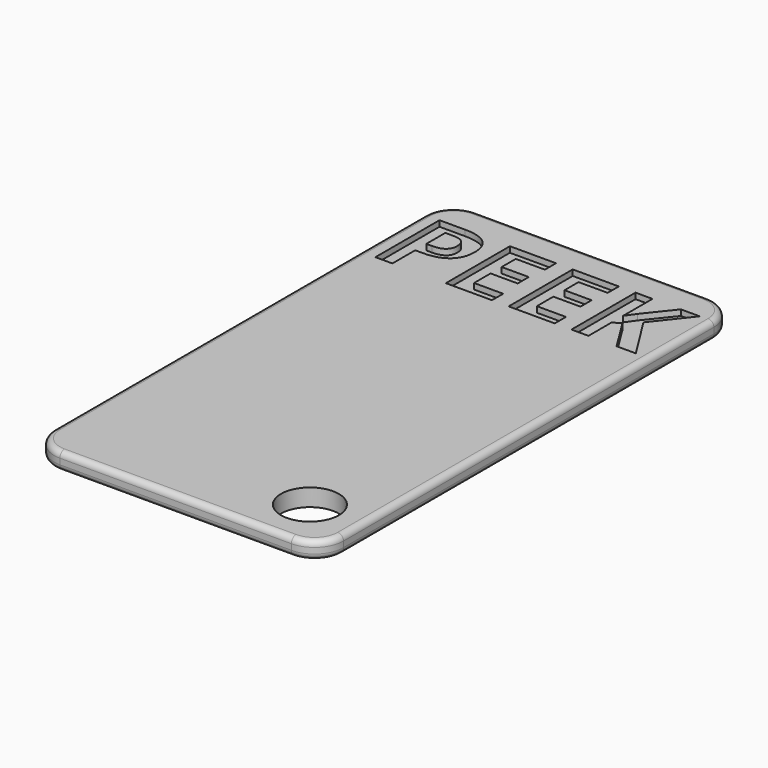
from build123d import *

# Parameters (mm, degrees)
F0_W         = 90
F0_H         = 50
F1_DEPTH     = 3
F2_R         = 1
F3_T1_DEPTH  = 3
F3_T4_ANGLE  = 90
F3_T6_ANGLE  = 90
F3_T8_ANGLE  = 90
F3_T10_ANGLE = 90
F3_T12_ANGLE = 90
F3_T14_ANGLE = 90
F3_T16_ANGLE = 90
F3_T18_ANGLE = 90
F5_ANGLE     = 90
F6_TEXT_SIZE = 19.3792581378
F7_DEPTH     = 1
F8_R         = 5
F9_DEPTH     = 3


# Not quite as in the source:
# - a fillet or chamfer that OpenCascade refuses, or shapes differently, is made with other operations: its cross-section is extruded or revolved along the edge and cut away or added
# - Text() gives the source's letters only with a copy of the font that has no kerning and outlines rounded to 1/6400 em; it was checked with that copy


with BuildPart() as f1:
    # F0 (on Top) → F1 (new body)
    with BuildSketch(Plane.XY):
        Rectangle(F0_W, F0_H)
    extrude(amount=F1_DEPTH)

    # F2
    f2_edges = [f1.edges().sort_by_distance(p)[0] for p in [
        (0, 25, 3),
        (-45, 0, 3),
        (0, -25, 3),
        (45, 0, 3),
        (0, 25, 0),
        (-45, 0, 0),
        (0, -25, 0),
        (45, 0, 0),
    ]]
    fillet(f2_edges, radius=F2_R)

    # F3: fillet of radius 5 on 4 edges, made by hand

    # F3_s2 → F3_t1 (cut)
    with BuildSketch(Plane.XY):
        with BuildLine():
            ThreePointArc((45, -20), (43.5355339059, -23.5355339059), (40, -25))
            Line((40, -25), (45, -25))
            Line((45, -25), (45, -20))
        make_face()
        with BuildLine():
            ThreePointArc((40, 25), (43.5355339059, 23.5355339059), (45, 20))
            Line((45, 20), (45, 25))
            Line((45, 25), (40, 25))
        make_face()
        with BuildLine():
            ThreePointArc((-40, 25), (-43.5355339059, 23.5355339059), (-45, 20))
            Line((-45, 20), (-45, 25))
            Line((-45, 25), (-40, 25))
        make_face()
        with BuildLine():
            ThreePointArc((-45, -20), (-43.5355339059, -23.5355339059), (-40, -25))
            Line((-40, -25), (-45, -25))
            Line((-45, -25), (-45, -20))
        make_face()
    extrude(amount=F3_T1_DEPTH, mode=Mode.SUBTRACT)

    # F3_s3 → F3_t4 (revolve, cut)
    with BuildSketch(Plane.YZ.offset(-40)):
        with BuildLine():
            ThreePointArc((-24, 0), (-24.7071067812, 0.2928932188), (-25, 1))
            Line((-25, 1), (-25, 0))
            Line((-25, 0), (-24, 0))
        make_face()
    revolve(axis=Axis((-40, -20, 0), (0, 0, -1)), revolution_arc=F3_T4_ANGLE, mode=Mode.SUBTRACT)

    # F3_s5 → F3_t6 (revolve, cut)
    with BuildSketch(Plane.XZ.offset(20)):
        with BuildLine():
            ThreePointArc((-44, 3), (-44.7071067812, 2.7071067812), (-45, 2))
            Line((-45, 2), (-45, 3))
            Line((-45, 3), (-44, 3))
        make_face()
    revolve(axis=Axis((-40, -20, 3), (0, 0, 1)), revolution_arc=F3_T6_ANGLE, mode=Mode.SUBTRACT)

    # F3_s7 → F3_t8 (revolve, cut)
    with BuildSketch(Plane.XZ.offset(-20)):
        with BuildLine():
            ThreePointArc((-44, 0), (-44.7071067812, 0.2928932188), (-45, 1))
            Line((-45, 1), (-45, 0))
            Line((-45, 0), (-44, 0))
        make_face()
    revolve(axis=Axis((-40, 20, 0), (0, 0, -1)), revolution_arc=F3_T8_ANGLE, mode=Mode.SUBTRACT)

    # F3_s9 → F3_t10 (revolve, cut)
    with BuildSketch(Plane.YZ.offset(-40)):
        with BuildLine():
            ThreePointArc((24, 3), (24.7071067812, 2.7071067812), (25, 2))
            Line((25, 2), (25, 3))
            Line((25, 3), (24, 3))
        make_face()
    revolve(axis=Axis((-40, 20, 3), (0, 0, 1)), revolution_arc=F3_T10_ANGLE, mode=Mode.SUBTRACT)

    # F3_s11 → F3_t12 (revolve, cut)
    with BuildSketch(Plane.YZ.offset(40)):
        with BuildLine():
            ThreePointArc((24, 0), (24.7071067812, 0.2928932188), (25, 1))
            Line((25, 1), (25, 0))
            Line((25, 0), (24, 0))
        make_face()
    revolve(axis=Axis((40, 20, 0), (0, 0, -1)), revolution_arc=F3_T12_ANGLE, mode=Mode.SUBTRACT)

    # F3_s13 → F3_t14 (revolve, cut)
    with BuildSketch(Plane.XZ.offset(-20)):
        with BuildLine():
            ThreePointArc((44, 3), (44.7071067812, 2.7071067812), (45, 2))
            Line((45, 2), (45, 3))
            Line((45, 3), (44, 3))
        make_face()
    revolve(axis=Axis((40, 20, 3), (0, 0, 1)), revolution_arc=F3_T14_ANGLE, mode=Mode.SUBTRACT)

    # F3_s15 → F3_t16 (revolve, cut)
    with BuildSketch(Plane.XZ.offset(20)):
        with BuildLine():
            ThreePointArc((44, 0), (44.7071067812, 0.2928932188), (45, 1))
            Line((45, 1), (45, 0))
            Line((45, 0), (44, 0))
        make_face()
    revolve(axis=Axis((40, -20, 0), (0, 0, -1)), revolution_arc=F3_T16_ANGLE, mode=Mode.SUBTRACT)

    # F3_s17 → F3_t18 (revolve, cut)
    with BuildSketch(Plane.YZ.offset(40)):
        with BuildLine():
            ThreePointArc((-24, 3), (-24.7071067812, 2.7071067812), (-25, 2))
            Line((-25, 2), (-25, 3))
            Line((-25, 3), (-24, 3))
        make_face()
    revolve(axis=Axis((40, -20, 3), (0, 0, 1)), revolution_arc=F3_T18_ANGLE, mode=Mode.SUBTRACT)


with BuildPart() as f1_1:
    # F5: moved
    add(f1.part.rotate(Axis((0, 0, 16.4477843791), (0, 0, 1)), F5_ANGLE))

    # F6 (on face) → F7 (cut)
    with BuildSketch(Plane.XY.offset(3)):
        with Locations((-24, 25.9722985371)):
            Text('PEEK', F6_TEXT_SIZE, font='Open Sans', font_style=FontStyle.BOLD, text_align=(TextAlign.LEFT, TextAlign.BOTTOM))
    extrude(amount=-F7_DEPTH, mode=Mode.SUBTRACT)

    # F8 (on face) → F9 (cut)
    with BuildSketch(Plane.XY.offset(3)):
        with Locations((16, -36)):
            Circle(F8_R)
    extrude(amount=-F9_DEPTH, mode=Mode.SUBTRACT)


solid = f1_1.part
